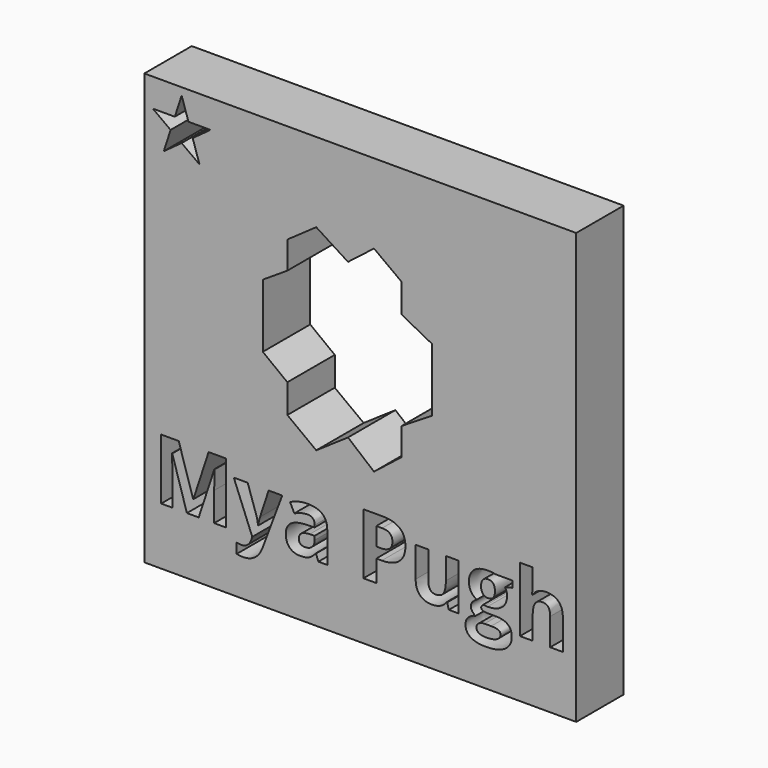
from build123d import *

# Parameters (mm, degrees)
F1_DEPTH     = 12.7
F2_TEXT_SIZE = 18.2446689113
F3_DEPTH     = 25.4


# Not quite as in the source:
# - Text() gives the source's letters only with a copy of the font that has no kerning and outlines rounded to 1/6400 em; it was checked with that copy


with BuildPart() as f1:
    # F0 (on Front) → F1 (new body)
    with BuildSketch(Plane.XZ):
        Polygon((-18.2614699006, 7.8926691785), (-12.9996910691, 11.2973507494), (-12.9996910691, 17.1781629324), (-6.809361279, 21.5113926679), (0, 17.1781629324), (0, 38.5347977281), (-43.64182055, 38.5347977281), (-43.64182055, 0), (-18.2614699006, 0), (-18.2614699006, 1.0833074339), align=None)
        Polygon((-37.1133275773, 32.4933745699), (-35.6531068683, 36.9874718067), (-34.1928861592, 32.4933745699), (-29.4675126827, 32.4933745699), (-33.29042013, 29.7158697288), (-31.8301994209, 25.2217724919), (-35.6531068683, 27.999277333), (-39.4760143156, 25.2217724919), (-38.0157936066, 29.7158697288), (-41.8387010539, 32.4933745699), align=None, mode=Mode.SUBTRACT)
        Polygon((0, 38.5347977281), (0, 17.1781629324), (5.5712950416, 21.5113926679), (11.4521095529, 17.1781629324), (11.4521095529, 10.9878340736), (17.9519522935, 7.5831529684), (17.9519522935, 0), (48.9035993814, 0), (48.9035993814, 38.5347977281), align=None)
        Polygon((-18.2614699006, -5.7260543108), (-18.2614699006, 0), (-43.64182055, 0), (-43.64182055, -53.7011027336), (0, -53.7011027336), (0, -15.9400962293), (-6.809361279, -20.5828435719), (-12.9996910691, -15.9400962293), (-12.9996910691, -9.7497683018), align=None)
        Polygon((48.9035993814, -53.7011027336), (48.9035993814, 0), (17.9519522935, 0), (17.9519522935, -6.0355709866), (11.4521095529, -10.0592849776), (11.4521095529, -15.9400962293), (5.5712950416, -20.5828435719), (0, -15.9400962293), (0, -53.7011027336), align=None)
    extrude(amount=F1_DEPTH)

    # F2 (on face) → F3 (cut)
    with BuildSketch(Plane.XZ.offset(12.7)):
        with Locations((-41.6775085032, -41.4349736032)):
            Text('Mya Pugh', F2_TEXT_SIZE, font='Open Sans', font_style=FontStyle.BOLD, text_align=(TextAlign.LEFT, TextAlign.BOTTOM))
    extrude(amount=-F3_DEPTH, mode=Mode.SUBTRACT)


solid = f1.part
